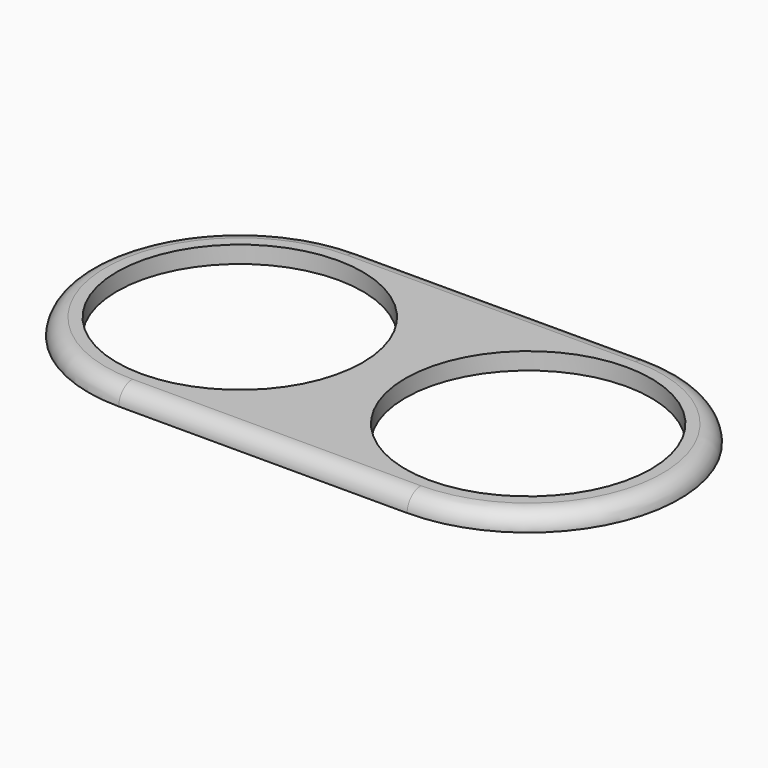
from build123d import *

# Parameters (mm, degrees)
F1_DEPTH = 7.62
F2_R     = 7.61999


# Not quite as in the source:
# - a fillet or chamfer is up to 0.001 mm smaller than in the source, because OpenCascade refuses the exact size


with BuildPart() as f1:
    # F0 (on Top) → F1 (new body)
    with BuildSketch(Plane.XY):
        with BuildLine():
            ThreePointArc((64.2620003332, -67.437), (131.6990003332, 0), (64.2620003332, 67.437))
            Line((64.2620003332, 67.437), (-64.2620003332, 67.437))
            ThreePointArc((-64.2620003332, 67.437), (-131.6990003332, 0), (-64.2620003332, -67.437))
            Line((-64.2620003332, -67.437), (64.2620003332, -67.437))
        make_face()
        with BuildLine():
            Line((-64.2620003332, 54.737), (64.2620003332, 54.737))
            ThreePointArc((64.2620003332, 54.737), (118.9990003332, 0), (64.2620003332, -54.737))
            Line((64.2620003332, -54.737), (-64.2620003332, -54.737))
            ThreePointArc((-64.2620003332, -54.737), (-118.9990003332, 0), (-64.2620003332, 54.737))
        make_face(mode=Mode.SUBTRACT)
        with BuildLine():
            ThreePointArc((64.2620003332, -54.737), (9.5250003332, 0), (64.2620003332, 54.737))
            Line((64.2620003332, 54.737), (-64.2620003332, 54.737))
            ThreePointArc((-64.2620003332, 54.737), (-9.5250003332, 0), (-64.2620003332, -54.737))
            Line((-64.2620003332, -54.737), (64.2620003332, -54.737))
        make_face()
    extrude(amount=F1_DEPTH)

    # F2 (radius 7.62 in the source; OpenCascade refuses exactly that, so slightly less here)
    f2_edges = [f1.edges().sort_by_distance(p)[0] for p in [
        (-131.699, 0, 7.62),
    ]]
    fillet(f2_edges, radius=F2_R)


solid = f1.part
